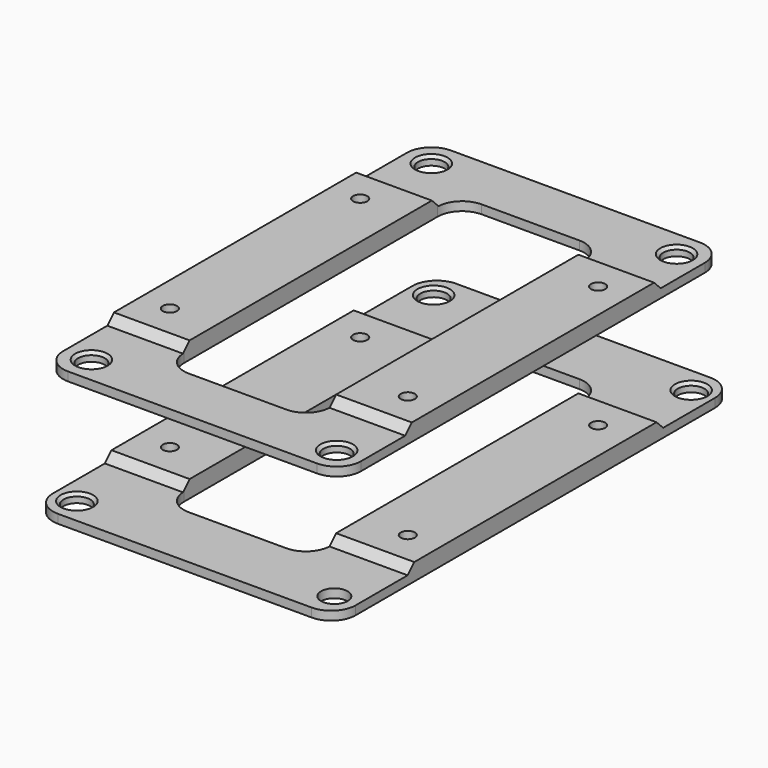
from build123d import *

# Parameters (mm, degrees)
F1_R      = 2.725
F3_DEPTH  = 1.8
F2_R      = 2.725
F1_W      = 16
F1_H      = 62
F1_R_2    = 1.45
F4_DEPTH  = 3.5
F2_W      = 15.5
F2_H      = 62
F2_R_2    = 1.45
F5_SIZE   = 1.69999
F5_2_SIZE = 1.69999
F6_R      = 5
F6_2_R    = 5
F7_SIZE   = 0.6
F7_2_SIZE = 0.6


# Not quite as in the source:
# - a fillet or chamfer is up to 0.001 mm smaller than in the source, because OpenCascade refuses the exact size


with BuildPart() as f3:
    # F1 (on Top) → F3 (new body)
    with BuildSketch(Plane.XY):
        Polygon((-15, -31), (-31, -31), (-31, -51), (31, -51), (31, -31), (15, -31), (15, -37.5), (-15, -37.5), align=None)
        with Locations((-26.3625, -45.6611894145)):
            Circle(F1_R, mode=Mode.SUBTRACT)
        with Locations((26.3625, -45.6611894145)):
            Circle(F1_R, mode=Mode.SUBTRACT)
    extrude(amount=F3_DEPTH)



with BuildPart() as f3b:
    # F1 (on Top) → F3, piece 2 (new body)
    with BuildSketch(Plane.XY):
        Polygon((31, 51), (-31, 51), (-31, 31), (-15, 31), (-15, 37.5), (15, 37.5), (15, 31), (31, 31), align=None)
        with Locations((-26.3625, 45.6611894145)):
            Circle(F1_R, mode=Mode.SUBTRACT)
        with Locations((26.3625, 45.6611894145)):
            Circle(F1_R, mode=Mode.SUBTRACT)
    extrude(amount=F3_DEPTH)


with BuildPart() as f3c:
    # F2 (on offset) → F3, piece 3 (new body)
    with BuildSketch(Plane.XY.offset(25)):
        Polygon((-15, -31), (-30.5, -31), (-30.5, -49), (30.5, -49), (30.5, -31), (15, -31), (15, -37.5), (-15, -37.5), align=None)
        with Locations((-25.1125, -43.4961259051)):
            Circle(F2_R, mode=Mode.SUBTRACT)
        with Locations((25.1125, -43.4961259051)):
            Circle(F2_R, mode=Mode.SUBTRACT)
    extrude(amount=F3_DEPTH)



with BuildPart() as f3d:
    # F2 (on offset) → F3, piece 4 (new body)
    with BuildSketch(Plane.XY.offset(25)):
        Polygon((30.5, 49), (-30.5, 49), (-30.5, 31), (-15, 31), (-15, 37.5), (15, 37.5), (15, 31), (30.5, 31), align=None)
        with Locations((-25.1125, 43.4961259051)):
            Circle(F2_R, mode=Mode.SUBTRACT)
        with Locations((25.1125, 43.4961259051)):
            Circle(F2_R, mode=Mode.SUBTRACT)
    extrude(amount=F3_DEPTH)


with BuildPart() as f3_1:
    add(f3.part)

    add(f3b.part)  # F4 merges F3b
    # F1 (on Top) → F4 (join)
    with BuildSketch(Plane.XY):
        with Locations((-23, 0)):
            Rectangle(F1_W, F1_H)
        with Locations((-24.3598286119, -24.3598286119)):
            Circle(F1_R_2, mode=Mode.SUBTRACT)
        with Locations((-24.3598622407, 24.3598622407)):
            Circle(F1_R_2, mode=Mode.SUBTRACT)
        with Locations((23, 0)):
            Rectangle(F1_W, F1_H)
        with Locations((24.3598286119, -24.3598286119)):
            Circle(F1_R_2, mode=Mode.SUBTRACT)
        with Locations((24.3598622407, 24.3598622407)):
            Circle(F1_R_2, mode=Mode.SUBTRACT)
    extrude(amount=F4_DEPTH)

    # F5 (size 1.7 in the source; OpenCascade refuses exactly that, so slightly less here)
    f5_edges = [f3_1.edges().sort_by_distance(p)[0] for p in [
        (-23, -31, 1.8),
        (23, -31, 1.8),
        (-23, 31, 1.8),
        (23, 31, 1.8),
    ]]
    chamfer(f5_edges, length=F5_SIZE)

    # F6#2
    f6_2_edges = [f3_1.edges().sort_by_distance(p)[0] for p in [
        (-15, 37.5, 0.9),
        (15, 37.5, 0.9),
        (31, -51, 0.9),
        (-31, -51, 0.9),
        (31, 51, 0.9),
        (-15, -37.5, 0.9),
        (15, -37.5, 0.9),
        (-31, 51, 0.9),
    ]]
    fillet(f6_2_edges, radius=F6_2_R)

    # F7
    f7_edges = [f3_1.edges().sort_by_distance(p)[0] for p in [
        (23.6375, 45.661189, 1.8),
        (-29.0875, 45.661189, 1.8),
        (-29.0875, -45.661189, 1.8),
    ]]
    chamfer(f7_edges, length=F7_SIZE)


with BuildPart() as f3c_1:
    add(f3c.part)

    add(f3d.part)  # F4#2 merges F3d
    # F2 (on offset) → F4, piece 2 (join)
    with BuildSketch(Plane.XY.offset(25)):
        with Locations((22.75, 0)):
            Rectangle(F2_W, F2_H)
        with Locations((24.3598286119, -24.3598286119)):
            Circle(F2_R_2, mode=Mode.SUBTRACT)
        with Locations((24.3598622407, 24.3598622407)):
            Circle(F2_R_2, mode=Mode.SUBTRACT)
        with Locations((-22.75, 0)):
            Rectangle(F2_W, F2_H)
        with Locations((-24.3598286119, -24.3598286119)):
            Circle(F2_R_2, mode=Mode.SUBTRACT)
        with Locations((-24.3598622407, 24.3598622407)):
            Circle(F2_R_2, mode=Mode.SUBTRACT)
    extrude(amount=F4_DEPTH)

    # F5#2 (size 1.7 in the source; OpenCascade refuses exactly that, so slightly less here)
    f5_2_edges = [f3c_1.edges().sort_by_distance(p)[0] for p in [
        (-22.75, -31, 26.8),
        (22.75, -31, 26.8),
        (-22.75, 31, 26.8),
        (22.75, 31, 26.8),
    ]]
    chamfer(f5_2_edges, length=F5_2_SIZE)

    # F6
    f6_edges = [f3c_1.edges().sort_by_distance(p)[0] for p in [
        (30.5, -49, 25.9),
        (-30.5, -49, 25.9),
        (15, 37.5, 25.9),
        (-15, 37.5, 25.9),
        (30.5, 49, 25.9),
        (-15, -37.5, 25.9),
        (15, -37.5, 25.9),
        (-30.5, 49, 25.9),
    ]]
    fillet(f6_edges, radius=F6_R)

    # F7#2
    f7_2_edges = [f3c_1.edges().sort_by_distance(p)[0] for p in [
        (-27.8375, 43.496126, 26.8),
        (22.3875, 43.496126, 26.8),
        (22.3875, -43.496126, 26.8),
        (-27.8375, -43.496126, 26.8),
    ]]
    chamfer(f7_2_edges, length=F7_2_SIZE)


solid = Compound([f3_1.part, f3c_1.part])
